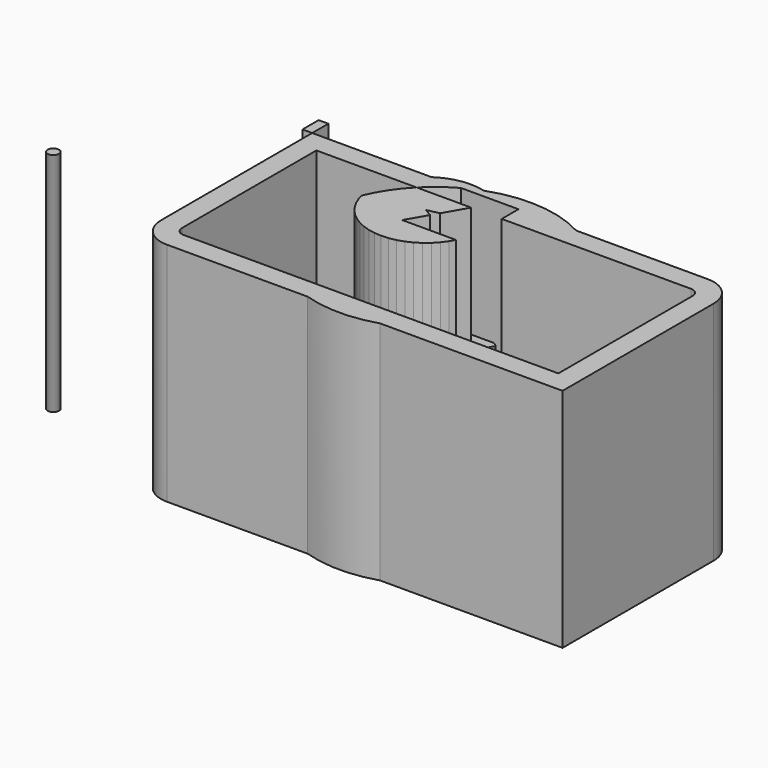
from build123d import *

# Parameters (mm, degrees)
F1_DEPTH = 25.4
F0_W     = 2.9361471534
F0_H     = 3.0584856868
F2_DEPTH = 25.4
F3_DEPTH = 68.58
F4_DEPTH = 30.48


# Not quite as in the source:
# - the program builds the solid bodies; features that only make, move or delete a surface that nothing else refers to are left out


with BuildPart() as f1:
    # F0 (on Top) → F1 (new body)
    with BuildSketch(Plane.XY):
        Polygon((-62.5154599547, 0), (-56.1654599547, 0), (-56.1654599547, 25.3359185696), (-31.9179130904, 25.3359185696), (-31.1432781089, 26.7449743701), (-29.895510103, 28.4623796944), (-28.4423331579, 30.0098559658), (-26.8066647421, 31.3629985591), (-26.2978242266, 31.6859185696), (-62.5154599547, 31.6859185696), align=None)
    extrude(amount=F1_DEPTH)

    # F0 (on Top) → F2 (join)
    with BuildSketch(Plane.XY):
        with BuildLine():
            Line((0, 25.3359185696), (25.8161057919, 25.3359185696))
            ThreePointArc((25.8161057919, 25.3359185696), (21.8631038448, 28.8163977328), (17.4465656341, 31.6859185696))
            Line((17.4465656341, 31.6859185696), (0, 31.6859185696))
            Line((0, 31.6859185696), (0, 25.3359185696))
        make_face()
        with BuildLine():
            ThreePointArc((17.4465656341, 31.6859185696), (21.8631038448, 28.8163977328), (25.8161057919, 25.3359185696))
            Line((25.8161057919, 25.3359185696), (57.3888527393, 25.3359185696))
            ThreePointArc((57.3888527393, 25.3359185696), (59.1849039635, 24.5919697938), (59.9288527393, 22.7959185696))
            Line((59.9288527393, 22.7959185696), (59.9288527393, 0))
            Line((59.9288527393, 0), (66.2788527393, 0))
            Line((66.2788527393, 0), (66.2788527393, 22.7959185696))
            ThreePointArc((66.2788527393, 22.7959185696), (63.6750320241, 29.0820978543), (57.3888527393, 31.6859185696))
            Line((57.3888527393, 31.6859185696), (17.4465656341, 31.6859185696))
        make_face()
        with BuildLine():
            Line((59.9288527393, -28.1205956364), (22.7510920415, -28.1205956364))
            ThreePointArc((22.7510920415, -28.1205956364), (17.1527881407, -31.8459094237), (10.9616661369, -34.4705956364))
            Line((10.9616661369, -34.4705956364), (66.2788527393, -34.4705956364))
            Line((66.2788527393, -34.4705956364), (66.2788527393, 0))
            Line((66.2788527393, 0), (59.9288527393, 0))
            Line((59.9288527393, 0), (59.9288527393, -28.1205956364))
        make_face()
        with BuildLine():
            ThreePointArc((10.9616661369, -34.4705956364), (17.1527881407, -31.8459094237), (22.7510920415, -28.1205956364))
            Line((22.7510920415, -28.1205956364), (0, -28.1205956364))
            Line((0, -28.1205956364), (0, -34.4705956364))
            Line((0, -34.4705956364), (10.9616661369, -34.4705956364))
        make_face()
        with BuildLine():
            Line((0, 31.6859185696), (17.4465656341, 31.6859185696))
            ThreePointArc((17.4465656341, 31.6859185696), (2.7670174678, 36.0655473043), (-12.4088213224, 33.9764807096))
            Line((-12.4088213224, 33.9764807096), (-10.6479057106, 33.404324544))
            Line((-10.6479057106, 33.404324544), (-8.727111947, 32.5004676073))
            Line((-8.727111947, 32.5004676073), (-7.4435880441, 31.6859185696))
            Line((-7.4435880441, 31.6859185696), (0, 31.6859185696))
        make_face()
        with Locations((-63.9835335314, 33.215161413)):
            Rectangle(F0_W, F0_H)
        with BuildLine():
            ThreePointArc((-10.9616661369, -34.4705956364), (0, -36.1715369873), (10.9616661369, -34.4705956364))
            Line((10.9616661369, -34.4705956364), (0, -34.4705956364))
            Line((0, -34.4705956364), (-10.9616661369, -34.4705956364))
        make_face()
        with BuildLine():
            Line((0, -34.4705956364), (0, -28.1205956364))
            Line((0, -28.1205956364), (-22.7510920415, -28.1205956364))
            ThreePointArc((-22.7510920415, -28.1205956364), (-17.1527881407, -31.8459094237), (-10.9616661369, -34.4705956364))
            Line((-10.9616661369, -34.4705956364), (0, -34.4705956364))
        make_face()
        with BuildLine():
            Line((-10.6479057106, 33.404324544), (-12.4088213224, 33.9764807096))
            ThreePointArc((-12.4088213224, 33.9764807096), (-14.9715630884, 32.9276841991), (-17.4465656341, 31.6859185696))
            Line((-17.4465656341, 31.6859185696), (-7.4435880441, 31.6859185696))
            Line((-7.4435880441, 31.6859185696), (-8.727111947, 32.5004676073))
            Line((-8.727111947, 32.5004676073), (-10.6479057106, 33.404324544))
        make_face()
        with BuildLine():
            ThreePointArc((-17.4465656341, 31.6859185696), (-14.9715630884, 32.9276841991), (-12.4088213224, 33.9764807096))
            Line((-12.4088213224, 33.9764807096), (-12.6668367542, 34.0603150054))
            Line((-12.6668367542, 34.0603150054), (-14.7520653292, 34.45809363))
            Line((-14.7520653292, 34.45809363), (-16.8707061353, 34.5913872114))
            Line((-16.8707061353, 34.5913872114), (-18.9893469415, 34.45809363))
            Line((-18.9893469415, 34.45809363), (-21.0745755165, 34.0603150054))
            Line((-21.0745755165, 34.0603150054), (-23.0935065601, 33.404324544))
            Line((-23.0935065601, 33.404324544), (-25.0143003236, 32.5004676073))
            Line((-25.0143003236, 32.5004676073), (-26.2978242266, 31.6859185696))
            Line((-26.2978242266, 31.6859185696), (-17.4465656341, 31.6859185696))
        make_face()
        with BuildLine():
            Line((-53.6254599547, -34.4705956364), (-10.9616661369, -34.4705956364))
            ThreePointArc((-10.9616661369, -34.4705956364), (-17.1527881407, -31.8459094237), (-22.7510920415, -28.1205956364))
            Line((-22.7510920415, -28.1205956364), (-53.6254599547, -28.1205956364))
            ThreePointArc((-53.6254599547, -28.1205956364), (-55.421511179, -27.3766468606), (-56.1654599547, -25.5805956364))
            Line((-56.1654599547, -25.5805956364), (-56.1654599547, 0))
            Line((-56.1654599547, 0), (-62.5154599547, 0))
            Line((-62.5154599547, 0), (-62.5154599547, -25.5805956364))
            ThreePointArc((-62.5154599547, -25.5805956364), (-59.9116392395, -31.8667749211), (-53.6254599547, -34.4705956364))
        make_face()
        Polygon((-62.5154599547, 0), (-56.1654599547, 0), (-56.1654599547, 25.3359185696), (-31.9179130904, 25.3359185696), (-31.1432781089, 26.7449743701), (-29.895510103, 28.4623796944), (-28.4423331579, 30.0098559658), (-26.8066647421, 31.3629985591), (-26.2978242266, 31.6859185696), (-62.5154599547, 31.6859185696), align=None)
        with BuildLine():
            ThreePointArc((-25.8161057919, 25.3359185696), (-21.8631038448, 28.8163977328), (-17.4465656341, 31.6859185696))
            Line((-17.4465656341, 31.6859185696), (-26.2978242266, 31.6859185696))
            Line((-26.2978242266, 31.6859185696), (-26.8066647421, 31.3629985591))
            Line((-26.8066647421, 31.3629985591), (-28.4423331579, 30.0098559658))
            Line((-28.4423331579, 30.0098559658), (-29.895510103, 28.4623796944))
            Line((-29.895510103, 28.4623796944), (-31.1432781089, 26.7449743701))
            Line((-31.1432781089, 26.7449743701), (-31.9179130904, 25.3359185696))
            Line((-31.9179130904, 25.3359185696), (-25.8161057919, 25.3359185696))
        make_face()
        with Locations((-63.9835335314, 36.2736470997)):
            Rectangle(F0_W, F0_H)
    extrude(amount=F2_DEPTH)

    # F0 (on Top) → F3, piece 2 (join)
    with BuildSketch(Plane.XY):
        with BuildLine():
            Line((0, 25.3359185696), (25.8161057919, 25.3359185696))
            ThreePointArc((25.8161057919, 25.3359185696), (21.8631038448, 28.8163977328), (17.4465656341, 31.6859185696))
            Line((17.4465656341, 31.6859185696), (0, 31.6859185696))
            Line((0, 31.6859185696), (0, 25.3359185696))
        make_face()
        with BuildLine():
            ThreePointArc((17.4465656341, 31.6859185696), (21.8631038448, 28.8163977328), (25.8161057919, 25.3359185696))
            Line((25.8161057919, 25.3359185696), (57.3888527393, 25.3359185696))
            ThreePointArc((57.3888527393, 25.3359185696), (59.1849039635, 24.5919697938), (59.9288527393, 22.7959185696))
            Line((59.9288527393, 22.7959185696), (59.9288527393, 0))
            Line((59.9288527393, 0), (66.2788527393, 0))
            Line((66.2788527393, 0), (66.2788527393, 22.7959185696))
            ThreePointArc((66.2788527393, 22.7959185696), (63.6750320241, 29.0820978543), (57.3888527393, 31.6859185696))
            Line((57.3888527393, 31.6859185696), (17.4465656341, 31.6859185696))
        make_face()
        with BuildLine():
            Line((59.9288527393, -28.1205956364), (22.7510920415, -28.1205956364))
            ThreePointArc((22.7510920415, -28.1205956364), (17.1527881407, -31.8459094237), (10.9616661369, -34.4705956364))
            Line((10.9616661369, -34.4705956364), (66.2788527393, -34.4705956364))
            Line((66.2788527393, -34.4705956364), (66.2788527393, 0))
            Line((66.2788527393, 0), (59.9288527393, 0))
            Line((59.9288527393, 0), (59.9288527393, -28.1205956364))
        make_face()
        with BuildLine():
            ThreePointArc((10.9616661369, -34.4705956364), (17.1527881407, -31.8459094237), (22.7510920415, -28.1205956364))
            Line((22.7510920415, -28.1205956364), (0, -28.1205956364))
            Line((0, -28.1205956364), (0, -34.4705956364))
            Line((0, -34.4705956364), (10.9616661369, -34.4705956364))
        make_face()
        with BuildLine():
            Line((0, 31.6859185696), (17.4465656341, 31.6859185696))
            ThreePointArc((17.4465656341, 31.6859185696), (2.7670174678, 36.0655473043), (-12.4088213224, 33.9764807096))
            Line((-12.4088213224, 33.9764807096), (-10.6479057106, 33.404324544))
            Line((-10.6479057106, 33.404324544), (-8.727111947, 32.5004676073))
            Line((-8.727111947, 32.5004676073), (-7.4435880441, 31.6859185696))
            Line((-7.4435880441, 31.6859185696), (0, 31.6859185696))
        make_face()
        with Locations((-63.9835335314, 33.215161413)):
            Rectangle(F0_W, F0_H)
        with BuildLine():
            ThreePointArc((-10.9616661369, -34.4705956364), (0, -36.1715369873), (10.9616661369, -34.4705956364))
            Line((10.9616661369, -34.4705956364), (0, -34.4705956364))
            Line((0, -34.4705956364), (-10.9616661369, -34.4705956364))
        make_face()
        with BuildLine():
            Line((0, -34.4705956364), (0, -28.1205956364))
            Line((0, -28.1205956364), (-22.7510920415, -28.1205956364))
            ThreePointArc((-22.7510920415, -28.1205956364), (-17.1527881407, -31.8459094237), (-10.9616661369, -34.4705956364))
            Line((-10.9616661369, -34.4705956364), (0, -34.4705956364))
        make_face()
        with BuildLine():
            Line((-10.6479057106, 33.404324544), (-12.4088213224, 33.9764807096))
            ThreePointArc((-12.4088213224, 33.9764807096), (-14.9715630884, 32.9276841991), (-17.4465656341, 31.6859185696))
            Line((-17.4465656341, 31.6859185696), (-7.4435880441, 31.6859185696))
            Line((-7.4435880441, 31.6859185696), (-8.727111947, 32.5004676073))
            Line((-8.727111947, 32.5004676073), (-10.6479057106, 33.404324544))
        make_face()
        with BuildLine():
            ThreePointArc((-17.4465656341, 31.6859185696), (-14.9715630884, 32.9276841991), (-12.4088213224, 33.9764807096))
            Line((-12.4088213224, 33.9764807096), (-12.6668367542, 34.0603150054))
            Line((-12.6668367542, 34.0603150054), (-14.7520653292, 34.45809363))
            Line((-14.7520653292, 34.45809363), (-16.8707061353, 34.5913872114))
            Line((-16.8707061353, 34.5913872114), (-18.9893469415, 34.45809363))
            Line((-18.9893469415, 34.45809363), (-21.0745755165, 34.0603150054))
            Line((-21.0745755165, 34.0603150054), (-23.0935065601, 33.404324544))
            Line((-23.0935065601, 33.404324544), (-25.0143003236, 32.5004676073))
            Line((-25.0143003236, 32.5004676073), (-26.2978242266, 31.6859185696))
            Line((-26.2978242266, 31.6859185696), (-17.4465656341, 31.6859185696))
        make_face()
        with BuildLine():
            Line((-53.6254599547, -34.4705956364), (-10.9616661369, -34.4705956364))
            ThreePointArc((-10.9616661369, -34.4705956364), (-17.1527881407, -31.8459094237), (-22.7510920415, -28.1205956364))
            Line((-22.7510920415, -28.1205956364), (-53.6254599547, -28.1205956364))
            ThreePointArc((-53.6254599547, -28.1205956364), (-55.421511179, -27.3766468606), (-56.1654599547, -25.5805956364))
            Line((-56.1654599547, -25.5805956364), (-56.1654599547, 0))
            Line((-56.1654599547, 0), (-62.5154599547, 0))
            Line((-62.5154599547, 0), (-62.5154599547, -25.5805956364))
            ThreePointArc((-62.5154599547, -25.5805956364), (-59.9116392395, -31.8667749211), (-53.6254599547, -34.4705956364))
        make_face()
        Polygon((-62.5154599547, 0), (-56.1654599547, 0), (-56.1654599547, 25.3359185696), (-31.9179130904, 25.3359185696), (-31.1432781089, 26.7449743701), (-29.895510103, 28.4623796944), (-28.4423331579, 30.0098559658), (-26.8066647421, 31.3629985591), (-26.2978242266, 31.6859185696), (-62.5154599547, 31.6859185696), align=None)
        with BuildLine():
            ThreePointArc((-25.8161057919, 25.3359185696), (-21.8631038448, 28.8163977328), (-17.4465656341, 31.6859185696))
            Line((-17.4465656341, 31.6859185696), (-26.2978242266, 31.6859185696))
            Line((-26.2978242266, 31.6859185696), (-26.8066647421, 31.3629985591))
            Line((-26.8066647421, 31.3629985591), (-28.4423331579, 30.0098559658))
            Line((-28.4423331579, 30.0098559658), (-29.895510103, 28.4623796944))
            Line((-29.895510103, 28.4623796944), (-31.1432781089, 26.7449743701))
            Line((-31.1432781089, 26.7449743701), (-31.9179130904, 25.3359185696))
            Line((-31.9179130904, 25.3359185696), (-25.8161057919, 25.3359185696))
        make_face()
        with Locations((-63.9835335314, 36.2736470997)):
            Rectangle(F0_W, F0_H)
        with BuildLine():
            ThreePointArc((-25.8161057919, 25.3359185696), (-30.1176460126, 20.0326604994), (-33.3458594379, 14.015482381))
            Line((-33.3458594379, 14.015482381), (-32.9474248719, 12.4636822018))
            Line((-32.9474248719, 12.4636822018), (-32.1659591287, 10.4899250394))
            Line((-32.1659591287, 10.4899250394), (-31.1432781089, 8.6296751702))
            Line((-31.1432781089, 8.6296751702), (-29.895510103, 6.9122698459))
            Line((-29.895510103, 6.9122698459), (-28.4423331579, 5.3647935745))
            Line((-28.4423331579, 5.3647935745), (-26.8066647421, 4.0116509812))
            Line((-26.8066647421, 4.0116509812), (-25.0143003236, 2.8741819331))
            Line((-25.0143003236, 2.8741819331), (-23.0935065601, 1.9703249963))
            Line((-23.0935065601, 1.9703249963), (-21.0745755165, 1.3143345349))
            Line((-21.0745755165, 1.3143345349), (-18.9893469415, 0.9165559103))
            Line((-18.9893469415, 0.9165559103), (-16.8707061353, 0.783262329))
            Line((-16.8707061353, 0.783262329), (-14.7520653292, 0.9165559103))
            Line((-14.7520653292, 0.9165559103), (-12.6668367542, 1.3143345349))
            Line((-12.6668367542, 1.3143345349), (-10.6479057106, 1.9703249963))
            Line((-10.6479057106, 1.9703249963), (-8.727111947, 2.8741819331))
            Line((-8.727111947, 2.8741819331), (-6.9347475286, 4.0116509812))
            Line((-6.9347475286, 4.0116509812), (-5.2990791128, 5.3647935745))
            Line((-5.2990791128, 5.3647935745), (-3.8459021677, 6.9122698459))
            Line((-3.8459021677, 6.9122698459), (-2.5981341618, 8.6296751702))
            Line((-2.5981341618, 8.6296751702), (-1.7600334856, 10.1541746408))
            Line((-1.7600334856, 10.1541746408), (-18.0142852782, 10.1541746408))
            Line((-18.0142852782, 10.1541746408), (-14.4664408012, 16.2992215323))
            Line((-14.4664408012, 16.2992215323), (-16.8707061353, 17.6873247702))
            Line((-16.8707061353, 17.6873247702), (-13.1839158222, 18.5206199579))
            Line((-13.1839158222, 18.5206199579), (-9.2491013341, 25.3359185696))
            Line((-9.2491013341, 25.3359185696), (-25.8161057919, 25.3359185696))
        make_face()
    extrude(amount=F3_DEPTH)


with BuildPart() as f2:
    # F0 (on Top) → F2, piece 2 (new body)
    with BuildSketch(Plane.XY):
        Polygon((-102.6427969337, -14.1767939518), (-102.6427969337, -13.9612792094), (-102.6698080932, -13.7474638651), (-102.7234044302, -13.5387199147), (-102.8027406983, -13.3383393748), (-102.9065657173, -13.1494823664), (-103.0332421045, -12.9751272773), (-103.1807720977, -12.8180237913), (-103.3468290607, -12.6806495244), (-103.5287941761, -12.5651709507), (-103.7237977452, -12.4734092363), (-103.9287644453, -12.4068115184), (-104.1404618291, -12.3664280827), (-104.3555513024, -12.3528958), (-104.5706407757, -12.3664280827), (-104.7823381595, -12.4068115184), (-104.9873048596, -12.4734092363), (-105.1823084288, -12.5651709507), (-105.3642735441, -12.6806495244), (-105.5303305072, -12.8180237913), (-105.6778605004, -12.9751272773), (-105.8045368876, -13.1494823664), (-105.9083619066, -13.3383393748), (-105.9876981747, -13.5387199147), (-106.0412945117, -13.7474638651), (-106.0683056712, -13.9612792094), (-106.0683056712, -14.1767939518), (-106.0412945117, -14.3906092961), (-105.9876981747, -14.5993532466), (-105.9083619066, -14.7997337864), (-105.8045368876, -14.9885907948), (-105.6778605004, -15.162945884), (-105.5303305072, -15.3200493699), (-105.3642735441, -15.4574236369), (-105.1823084288, -15.5729022106), (-104.9873048596, -15.6646639249), (-104.7823381595, -15.7312616428), (-104.5706407757, -15.7716450786), (-104.3555513024, -15.7851773612), (-104.1404618291, -15.7716450786), (-103.9287644453, -15.7312616428), (-103.7237977452, -15.6646639249), (-103.5287941761, -15.5729022106), (-103.3468290607, -15.4574236369), (-103.1807720977, -15.3200493699), (-103.0332421045, -15.162945884), (-102.9065657173, -14.9885907948), (-102.8027406983, -14.7997337864), (-102.7234044302, -14.5993532466), (-102.6698080932, -14.3906092961), align=None)
    extrude(amount=F2_DEPTH)

    # F0 (on Top) → F3 (join)
    with BuildSketch(Plane.XY):
        Polygon((-102.6427969337, -14.1767939518), (-102.6427969337, -13.9612792094), (-102.6698080932, -13.7474638651), (-102.7234044302, -13.5387199147), (-102.8027406983, -13.3383393748), (-102.9065657173, -13.1494823664), (-103.0332421045, -12.9751272773), (-103.1807720977, -12.8180237913), (-103.3468290607, -12.6806495244), (-103.5287941761, -12.5651709507), (-103.7237977452, -12.4734092363), (-103.9287644453, -12.4068115184), (-104.1404618291, -12.3664280827), (-104.3555513024, -12.3528958), (-104.5706407757, -12.3664280827), (-104.7823381595, -12.4068115184), (-104.9873048596, -12.4734092363), (-105.1823084288, -12.5651709507), (-105.3642735441, -12.6806495244), (-105.5303305072, -12.8180237913), (-105.6778605004, -12.9751272773), (-105.8045368876, -13.1494823664), (-105.9083619066, -13.3383393748), (-105.9876981747, -13.5387199147), (-106.0412945117, -13.7474638651), (-106.0683056712, -13.9612792094), (-106.0683056712, -14.1767939518), (-106.0412945117, -14.3906092961), (-105.9876981747, -14.5993532466), (-105.9083619066, -14.7997337864), (-105.8045368876, -14.9885907948), (-105.6778605004, -15.162945884), (-105.5303305072, -15.3200493699), (-105.3642735441, -15.4574236369), (-105.1823084288, -15.5729022106), (-104.9873048596, -15.6646639249), (-104.7823381595, -15.7312616428), (-104.5706407757, -15.7716450786), (-104.3555513024, -15.7851773612), (-104.1404618291, -15.7716450786), (-103.9287644453, -15.7312616428), (-103.7237977452, -15.6646639249), (-103.5287941761, -15.5729022106), (-103.3468290607, -15.4574236369), (-103.1807720977, -15.3200493699), (-103.0332421045, -15.162945884), (-102.9065657173, -14.9885907948), (-102.8027406983, -14.7997337864), (-102.7234044302, -14.5993532466), (-102.6698080932, -14.3906092961), align=None)
    extrude(amount=F3_DEPTH)


with BuildPart() as f4:
    # F0 (on Top) → F4 (new body)
    with BuildSketch(Plane.XY):
        with BuildLine():
            Line((-7.4435880441, 31.6859185696), (-17.4465656341, 31.6859185696))
            ThreePointArc((-17.4465656341, 31.6859185696), (-21.8631038448, 28.8163977328), (-25.8161057919, 25.3359185696))
            Line((-25.8161057919, 25.3359185696), (-9.2491013341, 25.3359185696))
            Line((-9.2491013341, 25.3359185696), (-6.1460616902, 30.7105408908))
            Line((-6.1460616902, 30.7105408908), (-6.9347475286, 31.3629985591))
            Line((-6.9347475286, 31.3629985591), (-7.4435880441, 31.6859185696))
        make_face()
    extrude(amount=F4_DEPTH)


solid = Compound([f1.part, f2.part, f4.part])
